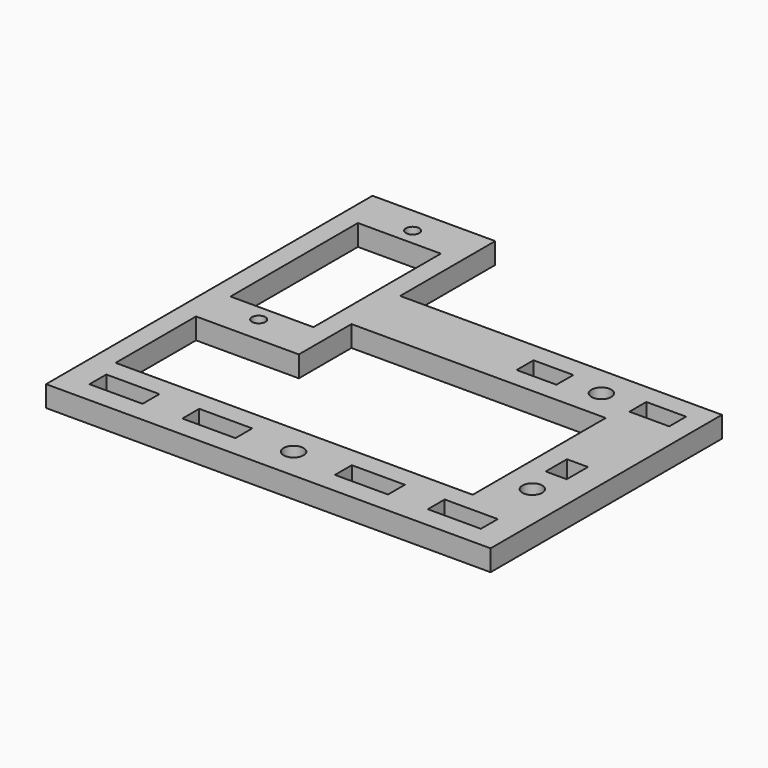
from build123d import *

# Parameters (mm, degrees)
F0_W     = 8
F0_H     = 3.175
F0_R     = 1
F0_R_2   = 1.5
F0_W_2   = 3.175
F0_H_2   = 4
F0_W_3   = 12.5
F0_H_3   = 24
F0_W_4   = 6
F1_DEPTH = 3.175


# Not quite as in the source:
# - a length typed as a fraction of an inch, garbled in the dataset ("3 / 203.2 mm" for 3/8 in), is restored


with BuildPart() as f1:
    # F0 (on Top) → F1 (new body)
    with BuildSketch(Plane.XY):
        Polygon((-41.0637862384, -14.8897265702), (-7.5637862384, -14.8897265702), (25.9362137616, -14.8897265702), (25.9362137616, 28.6977734298), (-22.5637862384, 28.6977734298), (-22.5637862384, 46.6102734298), (-41.0637862384, 46.6102734298), align=None)
        with Locations((-33.0637862384, -10.1272265702)):
            Rectangle(F0_W, F0_H, mode=Mode.SUBTRACT)
        with Locations((-19.0637862384, -10.1272265702)):
            Rectangle(F0_W, F0_H, mode=Mode.SUBTRACT)
        with Locations((-31.8137862384, 13.6102734298)):
            Circle(F0_R, mode=Mode.SUBTRACT)
        Polygon((15.7612137616, -5.5397265702), (-38.0637862384, -5.5397265702), (-38.0637862384, 9.6102734298), (-22.5637862384, 9.6102734298), (-22.5637862384, 19.5227734298), (15.7612137616, 19.5227734298), (15.7612137616, 9.6102734298), align=None, mode=Mode.SUBTRACT)
        with BuildLine():
            ThreePointArc((-7.5637862384, -11.6272265702), (-8.6244464102, -9.0665663985), (-6.0637862384, -10.1272265702))
            ThreePointArc((-6.0637862384, -10.1272265702), (-6.5031260667, -11.187886742), (-7.5637862384, -11.6272265702))
        make_face(mode=Mode.SUBTRACT)
        with Locations((3.9362137616, -10.1272265702)):
            Rectangle(F0_W, F0_H, mode=Mode.SUBTRACT)
        with Locations((17.9362137616, -10.1272265702)):
            Rectangle(F0_W, F0_H, mode=Mode.SUBTRACT)
        with Locations((20.3487137616, -0.0397265702)):
            Circle(F0_R_2, mode=Mode.SUBTRACT)
        with Locations((20.3487137616, 6.4602734298)):
            Rectangle(F0_W_2, F0_H_2, mode=Mode.SUBTRACT)
        with Locations((-31.8137862384, 28.1102734298)):
            Rectangle(F0_W_3, F0_H_3, mode=Mode.SUBTRACT)
        with Locations((-31.8137862384, 42.6102734298)):
            Circle(F0_R, mode=Mode.SUBTRACT)
        with Locations((2.9362137616, 24.1102734298)):
            Rectangle(F0_W_4, F0_H, mode=Mode.SUBTRACT)
        with Locations((11.4362137616, 24.1102734298)):
            Circle(F0_R_2, mode=Mode.SUBTRACT)
        with Locations((19.9362137616, 24.1102734298)):
            Rectangle(F0_W_4, F0_H, mode=Mode.SUBTRACT)
    extrude(amount=F1_DEPTH)


solid = f1.part
